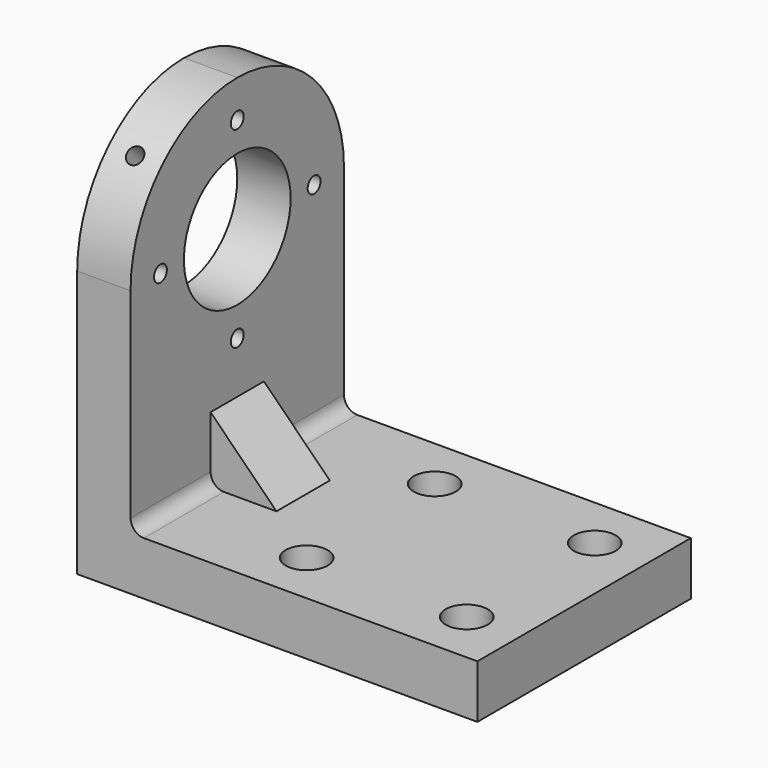
from build123d import *

# Parameters (mm, degrees)
F1_DEPTH  = 100
F2_R      = 99.99999
F3_R      = 8.75
F4_DEPTH  = 40.001
F3_R_2    = 15.75
F5_DEPTH  = 20
F6_R      = 50
F7_DEPTH  = 40.001
F11_DEPTH = 25
F12_R     = 10
F13_D     = 12.1
F16_D     = 12.1
F16_DEPTH = 69.85
F16_START = 0.1831763
F16_TIP   = 3.6352067451


# Not quite as in the source:
# - a fillet or chamfer is up to 0.001 mm smaller than in the source, because OpenCascade refuses the exact size


with BuildPart() as f1:
    # F0 (on Front) → F1 (new body, symmetric)
    with BuildSketch(Plane.XZ):
        Polygon((-72.2300410013, 0), (227.7699589987, 0), (227.7699589987, 40), (-32.2300410013, 40), (-32.2300410013, 300), (-72.2300410013, 300), align=None)
    extrude(amount=F1_DEPTH, both=True)

    # F2 (radius 100 in the source; OpenCascade refuses exactly that, so slightly less here)
    f2_edges = [f1.edges().sort_by_distance(p)[0] for p in [
        (-52.230041, -100, 300),
        (-52.230041, 100, 300),
    ]]
    fillet(f2_edges, radius=F2_R)

    # F3 (on face) → F4 (cut, through all)
    with BuildSketch(Plane.XY.offset(40)):
        with Locations((67.7699589987, 60)):
            Circle(F3_R)
        with Locations((187.7699589987, 60)):
            Circle(F3_R)
        with Locations((67.7699589987, -60)):
            Circle(F3_R)
        with Locations((187.7699589987, -60)):
            Circle(F3_R)
    extrude(amount=-F4_DEPTH, mode=Mode.SUBTRACT)

    # F3 (on face) → F5 (cut)
    with BuildSketch(Plane.XY.offset(40)):
        with Locations((187.7699589987, 60)):
            Circle(F3_R_2)
        with Locations((187.7699589987, 60)):
            Circle(F3_R, mode=Mode.SUBTRACT)
        with Locations((67.7699589987, 60)):
            Circle(F3_R_2)
        with Locations((67.7699589987, 60)):
            Circle(F3_R, mode=Mode.SUBTRACT)
        with Locations((67.7699589987, -60)):
            Circle(F3_R_2)
        with Locations((67.7699589987, -60)):
            Circle(F3_R, mode=Mode.SUBTRACT)
        with Locations((187.7699589987, -60)):
            Circle(F3_R_2)
        with Locations((187.7699589987, -60)):
            Circle(F3_R, mode=Mode.SUBTRACT)
    extrude(amount=-F5_DEPTH, mode=Mode.SUBTRACT)

    # F6 (on face) → F7 (cut, through all)
    with BuildSketch(Plane.YZ.offset(-32.2300410013)):
        with Locations((0, 200)):
            Circle(F6_R)
    extrude(amount=-F7_DEPTH, mode=Mode.SUBTRACT)

    # F10 (on offset) → F11 (join, symmetric)
    with BuildSketch(Plane(origin=(0, 0, 0), x_dir=(-1, 0, 0), z_dir=(0, 1, 0))):
        Polygon((-17.1466749161, 40), (32.2300410013, 40), (32.2300410013, 89.3767159174), align=None)
    extrude(amount=F11_DEPTH, both=True)

    # F12
    f12_edges = [f1.edges().sort_by_distance(p)[0] for p in [
        (-32.230041, 62.5, 40),
        (-32.230041, -62.5, 40),
    ]]
    fillet(f12_edges, radius=F12_R)

    # F13 (through all)
    with Locations(Plane.YZ.offset(-32.2300410013)):
        with Locations((0, 272), (72, 200), (0, 128), (-72, 200)):
            Hole(F13_D / 2)

    # F16
    # its depths count from where the whole tool has entered the part; down to there all is cleared
    with Locations(Plane(origin=(0, -170.7106781187, 170.7106781187), x_dir=(1, 0, 0), z_dir=(0, -0.7071067812, 0.7071067812)).offset(-F16_START)):
        with Locations((-52.2300410013, 141.4213562373)):
            Hole(F16_D / 2, depth=F16_DEPTH)
            with Locations((0, 0, -(F16_DEPTH + F16_TIP / 2))):  # 118° drill point
                Cone(0, F16_D / 2, F16_TIP, mode=Mode.SUBTRACT)


solid = f1.part
